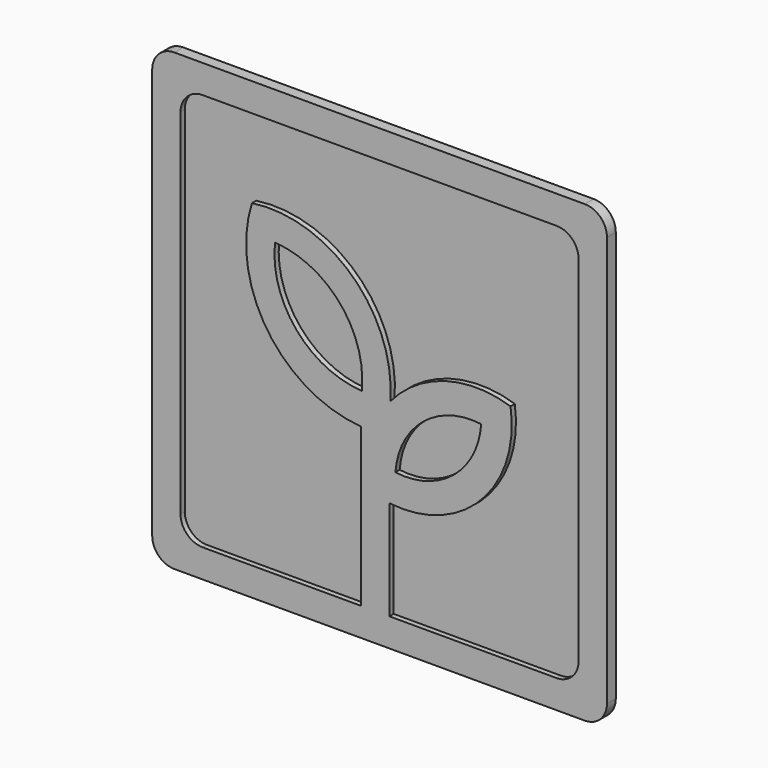
from build123d import *

# Parameters (mm, degrees)
F2_DEPTH = 1.651
F3_DEPTH = 3.175


# Not quite as in the source:
# - a feature of the source that left no trace in its solid (it failed there, or was rolled back) is left out


with BuildPart() as f2:
    # F0 (on Front) → F2 (new body)
    with BuildSketch(Plane.XZ):
        with BuildLine():
            Line((57.15, 63.5), (-57.15, 63.5))
            ThreePointArc((-57.15, 63.5), (-61.6401280605, 61.6401280605), (-63.5, 57.15))
            Line((-63.5, 57.15), (-63.5, -57.15))
            ThreePointArc((-63.5, -57.15), (-61.6401280605, -61.6401280605), (-57.15, -63.5))
            Line((-57.15, -63.5), (57.15, -63.5))
            ThreePointArc((57.15, -63.5), (61.6401280605, -61.6401280605), (63.5, -57.15))
            Line((63.5, -57.15), (63.5, 57.15))
            ThreePointArc((63.5, 57.15), (61.6401280605, 61.6401280605), (57.15, 63.5))
        make_face()
    extrude(amount=F2_DEPTH)

    # F1 (on face) → F3 (join)
    with BuildSketch(Plane.XZ):
        with BuildLine():
            Line((58.928, 65.278), (-58.928, 65.278))
            ThreePointArc((-58.928, 65.278), (-63.4181280605, 63.4181280605), (-65.278, 58.928))
            Line((-65.278, 58.928), (-65.278, -58.928))
            ThreePointArc((-65.278, -58.928), (-63.4181280605, -63.4181280605), (-58.928, -65.278))
            Line((-58.928, -65.278), (58.928, -65.278))
            ThreePointArc((58.928, -65.278), (63.4181280605, -63.4181280605), (65.278, -58.928))
            Line((65.278, -58.928), (65.278, 58.928))
            ThreePointArc((65.278, 58.928), (63.4181280605, 63.4181280605), (58.928, 65.278))
        make_face()
        with BuildLine():
            ThreePointArc((29.1683860123, 0), (21.2359008795, -15.4304684341), (4.5518055526, -20.1912078303))
            ThreePointArc((4.5518055526, -20.1912078303), (12.5076591177, -4.7892295638), (29.1683860123, 0))
        make_face(mode=Mode.SUBTRACT)
        with BuildLine():
            ThreePointArc((-30.0225467432, 26.633475086), (-11.3001914874, 17.269662026), (-5.1093608776, -2.7273676961))
            ThreePointArc((-5.1093608776, -2.7273676961), (-23.8921161087, 6.5851949341), (-30.0225467432, 26.633475086))
        make_face(mode=Mode.SUBTRACT)
        with BuildLine():
            Line((-5.3865113296, -11.8381703437), (-5.3865113296, -57.15))
            Line((-5.3865113296, -57.15), (-50.8, -57.15))
            ThreePointArc((-50.8, -57.15), (-55.2901280605, -55.2901280605), (-57.15, -50.8))
            Line((-57.15, -50.8), (-57.15, 50.8))
            ThreePointArc((-57.15, 50.8), (-55.2901280605, 55.2901280605), (-50.8, 57.15))
            Line((-50.8, 57.15), (50.8, 57.15))
            ThreePointArc((50.8, 57.15), (55.2901280605, 55.2901280605), (57.15, 50.8))
            Line((57.15, 50.8), (57.15, -50.8))
            ThreePointArc((57.15, -50.8), (55.2901280605, -55.2901280605), (50.8, -57.15))
            Line((50.8, -57.15), (2.8426104691, -57.15))
            Line((2.8426104691, -57.15), (2.8426104691, -28.5558674872))
            ThreePointArc((2.8426104691, -28.5558674872), (29.0723668952, -19.260680993), (37.6052677218, 7.2268673576))
            ThreePointArc((37.6052677218, 7.2268673576), (18.8257654598, 7.524261984), (3.0884773301, -2.7273676961))
            ThreePointArc((3.0884773301, -2.7273676961), (-7.830876963, 25.422268659), (-36.6427004337, 34.4507321715))
            ThreePointArc((-36.6427004337, 34.4507321715), (-32.213387286, 3.7443986853), (-5.3865113296, -11.8381703437))
        make_face(mode=Mode.SUBTRACT)
    extrude(amount=F3_DEPTH)


solid = f2.part
